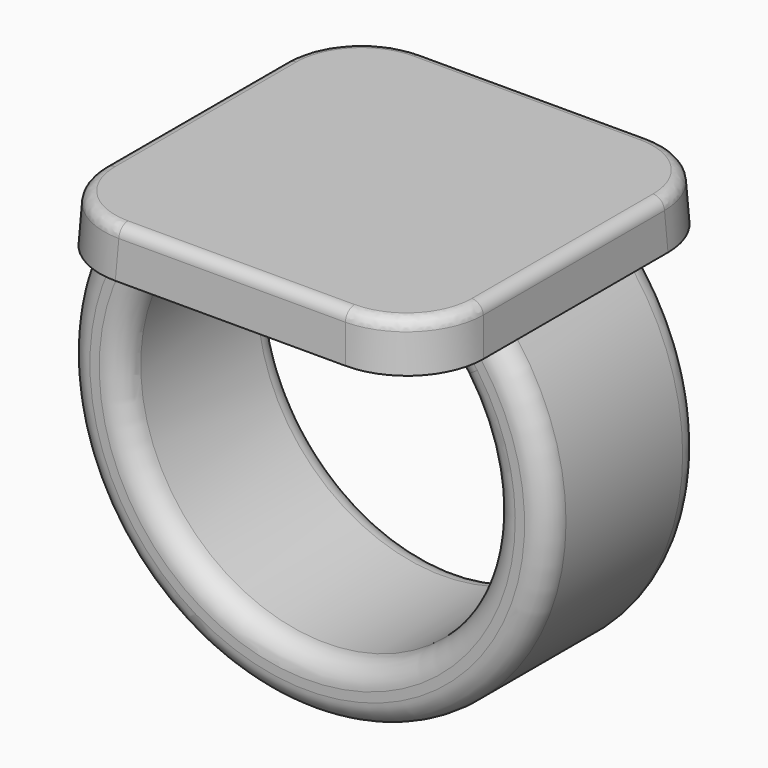
from build123d import *

# Parameters (mm, degrees)
F0_W          = 25.4
F0_H          = 25.4
F1_DEPTH      = 3.175
F1_TAPER      = 3
F3_W          = 5.08
F3_H          = 12.7
F6_DEPTH      = 6.35
F6_DEPTH_BACK = 6.35
F7_R          = 5.08
F8_R          = 1.524
F9_R          = 0.762


with BuildPart() as f1:
    # F0 (on Top) → F1 (new body)
    with BuildSketch(Plane.XY):
        Rectangle(F0_W, F0_H)
    extrude(amount=F1_DEPTH, taper=F1_TAPER)

    # F4: sweep along a path in F2
    with BuildLine(Plane.XZ) as f4_path:
        ThreePointArc((-10.16, 0), (0, -23.5582897328), (10.16, 0))
    # F3 (on face) → F4 (sweep)
    with BuildSketch(Plane(origin=(0, 0, 0), x_dir=(1, 0, 0), z_dir=(0, 0, -1))):
        with Locations((-10.16, 0)):
            Rectangle(F3_W, F3_H)
    sweep(path=f4_path.line)

    # F5 (on Front) → F6 (join, two sides)
    with BuildSketch(Plane.XZ) as f6_sk:
        with BuildLine():
            Line((10.0130578512, -2.535746045), (10.16, 0))
            Line((10.16, 0), (7.62, 0))
            ThreePointArc((7.62, 0), (8.9072265211, -1.1822790439), (10.0130578512, -2.535746045))
        make_face()
    extrude(amount=F6_DEPTH)
    extrude(f6_sk.sketch, amount=-F6_DEPTH_BACK)

    # F7
    f7_edges = [f1.edges().sort_by_distance(p)[0] for p in [
        (12.616803, 12.616803, 1.5875),
        (12.616803, -12.616803, 1.5875),
        (-12.616803, -12.616803, 1.5875),
        (-12.616803, 12.616803, 1.5875),
    ]]
    fillet(f7_edges, radius=F7_R)

    # F8
    f8_edges = [f1.edges().sort_by_distance(p)[0] for p in [
        (-1.743325, 6.35, -21.711017),
        (-1.743325, -6.35, -21.711017),
        (8.907227, -6.35, -1.182279),
        (0, -6.35, -25.501344),
        (0, 6.35, -25.501344),
        (8.907227, 6.35, -1.182279),
    ]]
    fillet(f8_edges, radius=F8_R)

    # F9
    f9_edges = [f1.edges().sort_by_distance(p)[0] for p in [
        (0, -12.533605, 3.175),
        (-11.048589, -11.048589, 3.175),
        (11.048589, -11.048589, 3.175),
        (-12.533605, 0, 3.175),
        (12.533605, 0, 3.175),
        (-11.048589, 11.048589, 3.175),
        (11.048589, 11.048589, 3.175),
        (0, 12.533605, 3.175),
    ]]
    fillet(f9_edges, radius=F9_R)


solid = f1.part
